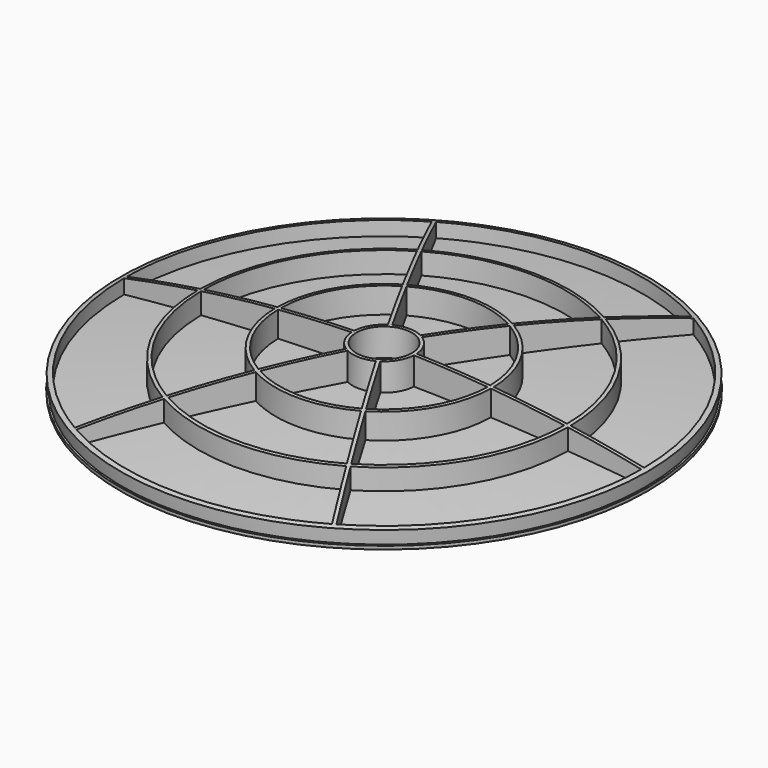
from build123d import *

# Parameters (mm, degrees)
F1_R            = 25.4
F3_REACH        = 113.1180489686
F5_REACH        = 291.4531103482
F5_COPIES_COUNT = 6


# Not quite as in the source:
# - a pattern or mirror of a feature is missing from the dataset's text; its kind, count and spacing are read off the source's solid


with BuildPart() as f2:
    # F0 (on Front) → F2 (revolve)
    with BuildSketch(Plane.XZ):
        with BuildLine():
            ThreePointArc((0, 15.875), (120.1471765301, 12.6933235295), (239.9575670804, 3.1572127131))
            Line((239.9575670804, 3.1572127131), (241.3, 15.7860635657))
            ThreePointArc((241.3, 15.7860635657), (121.3212428643, 34.8850889286), (0, 41.275))
            Line((0, 41.275), (0, 15.875))
        make_face()
    revolve(axis=Axis((0, 0, 0), (0, 0, 1)))

    f3_end = f2.faces().sort_by_distance((-121.3212428643, 0, 34.8850889286))[0]
    # F1 (on Top) → F3 (cut, up to a face of the model that its end follows)
    with BuildSketch(Plane.XY):
        Circle(F1_R)
    f3_long = extrude(amount=F3_REACH, mode=Mode.PRIVATE)
    add(split(f3_long, bisect_by=f3_end, keep=Keep.BOTTOM, mode=Mode.PRIVATE), mode=Mode.SUBTRACT)

    f5_end = f2.faces().sort_by_distance((-133.9444041338, 0, 33.4814561279))[0]
    # F4 (on Top) → F5 (cut, up to a face of the model that its end follows)
    with BuildSketch(Plane.XY):
        with BuildLine():
            Line((-83.3644585536, -147.5664777602), (-117.013807348, -205.8488595137))
            ThreePointArc((-117.013807348, -205.8488595137), (0, -236.7825670804), (117.013807348, -205.8488595137))
            Line((117.013807348, -205.8488595137), (83.3644585536, -147.5664777602))
            ThreePointArc((83.3644585536, -147.5664777602), (0, -169.4859826313), (-83.3644585536, -147.5664777602))
        make_face()
        with BuildLine():
            Line((-48.1275387874, -86.534342423), (-81.7768875818, -144.8167241765))
            ThreePointArc((-81.7768875818, -144.8167241765), (0, -166.3109826313), (81.7768875818, -144.8167241765))
            Line((81.7768875818, -144.8167241765), (48.1275387874, -86.534342423))
            ThreePointArc((48.1275387874, -86.534342423), (0, -99.0174348704), (-48.1275387874, -86.534342423))
        make_face()
        with BuildLine():
            Line((-12.8906190213, -25.5022070858), (-46.5399678156, -83.7845888393))
            ThreePointArc((-46.5399678156, -83.7845888393), (0, -95.8427145445), (46.5399678156, -83.7845888393))
            Line((46.5399678156, -83.7845888393), (12.8906190213, -25.5022070858))
            ThreePointArc((12.8906190213, -25.5022070858), (0, -28.575), (-12.8906190213, -25.5022070858))
        make_face()
    f5_long = extrude(amount=F5_REACH, mode=Mode.PRIVATE)
    f5 = split(f5_long, bisect_by=f5_end, keep=Keep.BOTTOM, mode=Mode.PRIVATE)
    add(f5, mode=Mode.SUBTRACT)

    # F5_copies: F5 ×6 about axis
    f5_copies_axis = Axis((0, 0, 0), (0, 0, 1))
    for i in range(1, F5_COPIES_COUNT):
        add(f5.rotate(f5_copies_axis, i * 360 / F5_COPIES_COUNT), mode=Mode.SUBTRACT)

    # F6 (on Front) → F7 (revolve)
    with BuildSketch(Plane.XZ):
        with BuildLine():
            Line((0, 15.875), (0, 12.7))
            ThreePointArc((0, 12.7), (120.8169896993, 9.5228042866), (241.3, 0))
            Line((241.3, 0), (241.6332872928, 3.1574585635))
            ThreePointArc((241.6332872928, 3.1574585635), (120.9838639945, 12.6934158948), (0, 15.875))
        make_face()
    revolve(axis=Axis((0, 0, 3.1572127131), (0, 0, 1)))


solid = f2.part
